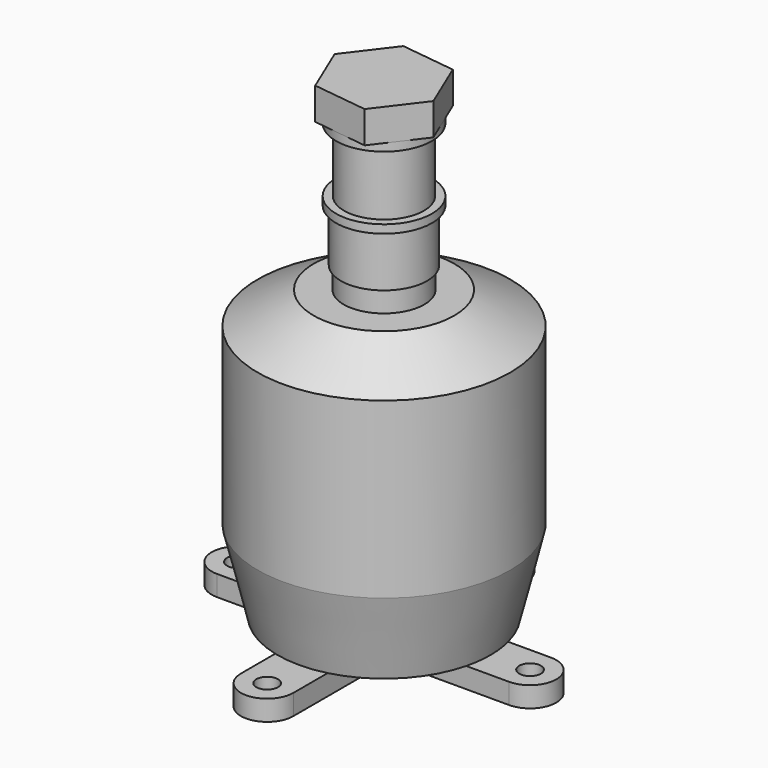
from build123d import *

# Parameters (mm, degrees)
F0_R      = 21.1455
F2_R      = 25.0825
F4_DEPTH  = 34.544
F6_R      = 13.97
F4_FACE_R = 25.0825
F8_R      = 8.001
F9_DEPTH  = 4.318
F10_R     = 3.00355
F11_DEPTH = 15.24
F12_R     = 6.0325
F13_DEPTH = 4.064
F14_R     = 2.9845
F15_DEPTH = 2.794
F16_R     = 2.15265
F17_DEPTH = 4.953
F18_R     = 2.15265
F18_R_2   = 7.0485
F19_DEPTH = 4.064
F20_R     = 8.5725
F21_DEPTH = 10.414
F22_R     = 9.525
F23_DEPTH = 1.651
F24_R     = 7.9375
F25_DEPTH = 12.7
F26_R     = 9.525
F27_DEPTH = 1.651
F29_DEPTH = 6.35


# Not quite as in the source:
# - a feature names something its author has since deleted; it is built from what else it names


with BuildPart() as f3:
    # F0 (on Top) → F3 section 0
    with BuildSketch(Plane.XY):
        Circle(F0_R)
    # F2 (on offset) → F3 section 1
    with BuildSketch(Plane.XY.offset(16.129)):
        Circle(F2_R)
    loft()

    # F4 (add): a face of the model
    f4_faces = [f3.faces().sort_by_distance(p)[0] for p in [
        (0, 0, 16.129),
    ]]
    extrude(f4_faces, amount=F4_DEPTH)

    # F6 (on offset) → F7 section 0
    with BuildSketch(Plane.XY.offset(57.023)):
        Circle(F6_R)
    # F4_face (on face) → F7 section 1
    with BuildSketch(Plane.XY.offset(50.673)):
        Circle(F4_FACE_R)
    loft()

    # F8 (on face) → F9 (join)
    with BuildSketch(Plane.XY.offset(57.023)):
        Circle(F8_R)
    extrude(amount=F9_DEPTH)

    # F10 (on face) → F11 (join)
    with BuildSketch(Plane.XY.offset(61.341)):
        Circle(F10_R)
    extrude(amount=F11_DEPTH)

    # F12 (on face) → F13 (join)
    with BuildSketch(Plane(origin=(0, 0, 0), x_dir=(1, 0, 0), z_dir=(0, 0, -1))):
        Circle(F12_R)
    extrude(amount=F13_DEPTH)

    # F14 (on face) → F15 (join)
    with BuildSketch(Plane(origin=(0, 0, -4.064), x_dir=(1, 0, 0), z_dir=(0, 0, -1))):
        Circle(F14_R)
    extrude(amount=F15_DEPTH)

    # F16 (on face) → F17 (cut)
    with BuildSketch(Plane(origin=(0, 0, 0), x_dir=(1, 0, 0), z_dir=(0, 0, -1))):
        with Locations((0, 13.26515)):
            Circle(F16_R)
        with Locations((13.26515, 0)):
            Circle(F16_R)
        with Locations((0, -13.26515)):
            Circle(F16_R)
        with Locations((-13.26515, 0)):
            Circle(F16_R)
    extrude(amount=-F17_DEPTH, mode=Mode.SUBTRACT)

    # F18 (on face) → F19 (join)
    with BuildSketch(Plane(origin=(0, 0, 0), x_dir=(1, 0, 0), z_dir=(0, 0, -1))):
        with BuildLine():
            ThreePointArc((11.557, 5.207), (7.0668719395, 7.0668719395), (5.207, 11.557))
            Line((5.207, 11.557), (5.207, 29.01315))
            ThreePointArc((5.207, 29.01315), (0, 34.22015), (-5.207, 29.01315))
            Line((-5.207, 29.01315), (-5.207, 11.557))
            ThreePointArc((-5.207, 11.557), (-7.0668719395, 7.0668719395), (-11.557, 5.207))
            Line((-11.557, 5.207), (-29.01315, 5.207))
            ThreePointArc((-29.01315, 5.207), (-34.22015, 0), (-29.01315, -5.207))
            Line((-29.01315, -5.207), (-11.557, -5.207))
            ThreePointArc((-11.557, -5.207), (-7.0668719395, -7.0668719395), (-5.207, -11.557))
            Line((-5.207, -11.557), (-5.207, -29.01315))
            ThreePointArc((-5.207, -29.01315), (0, -34.22015), (5.207, -29.01315))
            Line((5.207, -29.01315), (5.207, -11.557))
            ThreePointArc((5.207, -11.557), (7.0668719395, -7.0668719395), (11.557, -5.207))
            Line((11.557, -5.207), (29.01315, -5.207))
            ThreePointArc((29.01315, -5.207), (34.22015, 0), (29.01315, 5.207))
            Line((29.01315, 5.207), (11.557, 5.207))
        make_face()
        with Locations((0, -29.01315)):
            Circle(F18_R, mode=Mode.SUBTRACT)
        with Locations((0, -13.26515)):
            Circle(F18_R, mode=Mode.SUBTRACT)
        with Locations((-29.01315, 0)):
            Circle(F18_R, mode=Mode.SUBTRACT)
        with Locations((-13.26515, 0)):
            Circle(F18_R, mode=Mode.SUBTRACT)
        Circle(F18_R_2, mode=Mode.SUBTRACT)
        with Locations((13.26515, 0)):
            Circle(F18_R, mode=Mode.SUBTRACT)
        with Locations((0, 13.26515)):
            Circle(F18_R, mode=Mode.SUBTRACT)
        with Locations((29.01315, 0)):
            Circle(F18_R, mode=Mode.SUBTRACT)
        with Locations((0, 29.01315)):
            Circle(F18_R, mode=Mode.SUBTRACT)
    extrude(amount=F19_DEPTH)

    # F20 (on face) → F21 (join)
    with BuildSketch(Plane.XY.offset(61.341)):
        Circle(F20_R)
    extrude(amount=F21_DEPTH)

    # F22 (on face) → F23 (join)
    with BuildSketch(Plane.XY.offset(71.755)):
        Circle(F22_R)
    extrude(amount=F23_DEPTH)

    # F24 (on face) → F25 (join)
    with BuildSketch(Plane.XY.offset(73.406)):
        Circle(F24_R)
    extrude(amount=F25_DEPTH)

    # F26 (on face) → F27 (join)
    with BuildSketch(Plane.XY.offset(86.106)):
        Circle(F26_R)
    extrude(amount=F27_DEPTH)

    # F28 (on face) → F29 (join)
    with BuildSketch(Plane.XY.offset(87.757)):
        Polygon((6.6499638915, 8.760449774), (-4.2617901071, 10.1392625512), (-10.9117539986, 1.3788127773), (-6.6499638915, -8.760449774), (4.2617901071, -10.1392625512), (10.9117539986, -1.3788127773), align=None)
    extrude(amount=F29_DEPTH)


solid = f3.part
